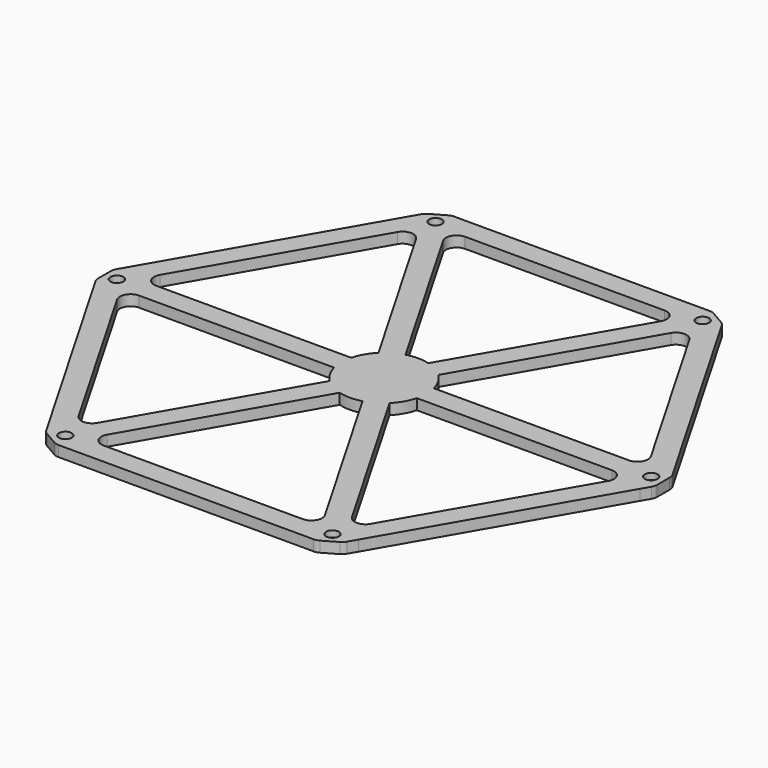
from build123d import *

# Parameters (mm, degrees)
F0_R     = 3
F1_DEPTH = 5
F2_DEPTH = 2
F3_R     = 5
F4_R     = 5
F0_R_2   = 15
F5_DEPTH = 5
F6_DEPTH = 5
F7_DEPTH = 3


# Not quite as in the source:
# - a feature names something its author has since deleted; it is built from what else it names


with BuildPart() as f1:
    # F0 (on Top) → F1 (new body)
    with BuildSketch(Plane.XY):
        Polygon((55.3523313466, 115.8730502097), (-55.3523313466, 115.8730502097), (-61.1258340385, 115.8730502097), (-69.7860880763, 110.8730502097), (-72.6728394223, 105.8730502097), (-128.0251707689, 10), (-130.9119221148, 5), (-130.9119221148, -5), (-128.0251707689, -10), (-72.6728394223, -105.8730502097), (-69.7860880763, -110.8730502097), (-61.1258340385, -115.8730502097), (-55.3523313466, -115.8730502097), (55.3523313466, -115.8730502097), (61.1258340385, -115.8730502097), (69.7860880763, -110.8730502097), (72.6728394223, -105.8730502097), (128.0251707689, -10), (130.9119221148, -5), (130.9119221148, 5), (128.0251707689, 10), (72.6728394223, 105.8730502097), (69.7860880763, 110.8730502097), (61.1258340385, 115.8730502097), align=None)
        with Locations((-62.5692097115, -108.3730502097)):
            Circle(F0_R, mode=Mode.SUBTRACT)
        with Locations((62.5692097115, -108.3730502097)):
            Circle(F0_R, mode=Mode.SUBTRACT)
        with Locations((-125.1384194229, 0)):
            Circle(F0_R, mode=Mode.SUBTRACT)
        Polygon((-119.364916731, -5), (-119.364916731, 0), (-119.364916731, 5), (-64.0125853844, 100.8730502097), (-59.6824583655, 103.3730502097), (-55.3523313466, 105.8730502097), (55.3523313466, 105.8730502097), (59.6824583655, 103.3730502097), (64.0125853844, 100.8730502097), (119.364916731, 5), (119.364916731, 0), (119.364916731, -5), (64.0125853844, -100.8730502097), (59.6824583655, -103.3730502097), (55.3523313466, -105.8730502097), (-55.3523313466, -105.8730502097), (-59.6824583655, -103.3730502097), (-64.0125853844, -100.8730502097), align=None, mode=Mode.SUBTRACT)
        with Locations((-62.5692097115, 108.3730502097)):
            Circle(F0_R, mode=Mode.SUBTRACT)
        with Locations((125.1384194229, 0)):
            Circle(F0_R, mode=Mode.SUBTRACT)
        with Locations((62.5692097115, 108.3730502097)):
            Circle(F0_R, mode=Mode.SUBTRACT)
        with BuildLine():
            Line((-59.6824583655, 103.3730502097), (-64.0125853844, 100.8730502097))
            Line((-64.0125853844, 100.8730502097), (-14.0125853844, 14.2705098312))
            ThreePointArc((-14.0125853844, 14.2705098312), (-10, 17.3205080757), (-5.3523313466, 19.2705098312))
            Line((-5.3523313466, 19.2705098312), (-55.3523313466, 105.8730502097))
            Line((-55.3523313466, 105.8730502097), (-59.6824583655, 103.3730502097))
        make_face()
        with BuildLine():
            Line((55.3523313466, 105.8730502097), (5.3523313466, 19.2705098312))
            ThreePointArc((5.3523313466, 19.2705098312), (10, 17.3205080757), (14.0125853844, 14.2705098312))
            Line((14.0125853844, 14.2705098312), (64.0125853844, 100.8730502097))
            Line((64.0125853844, 100.8730502097), (59.6824583655, 103.3730502097))
            Line((59.6824583655, 103.3730502097), (55.3523313466, 105.8730502097))
        make_face()
        with BuildLine():
            Line((119.364916731, 5), (19.364916731, 5))
            ThreePointArc((19.364916731, 5), (19.8405939253, 2.5200858497), (20, 0))
            ThreePointArc((20, 0), (19.8405939253, -2.5200858497), (19.364916731, -5))
            Line((19.364916731, -5), (119.364916731, -5))
            Line((119.364916731, -5), (119.364916731, 0))
            Line((119.364916731, 0), (119.364916731, 5))
        make_face()
        with BuildLine():
            ThreePointArc((14.0125853844, -14.2705098312), (10, -17.3205080757), (5.3523313466, -19.2705098312))
            Line((5.3523313466, -19.2705098312), (55.3523313466, -105.8730502097))
            Line((55.3523313466, -105.8730502097), (59.6824583655, -103.3730502097))
            Line((59.6824583655, -103.3730502097), (64.0125853844, -100.8730502097))
            Line((64.0125853844, -100.8730502097), (14.0125853844, -14.2705098312))
        make_face()
        with BuildLine():
            Line((-14.0125853844, -14.2705098312), (-64.0125853844, -100.8730502097))
            Line((-64.0125853844, -100.8730502097), (-59.6824583655, -103.3730502097))
            Line((-59.6824583655, -103.3730502097), (-55.3523313466, -105.8730502097))
            Line((-55.3523313466, -105.8730502097), (-5.3523313466, -19.2705098312))
            ThreePointArc((-5.3523313466, -19.2705098312), (-10, -17.3205080757), (-14.0125853844, -14.2705098312))
        make_face()
        with BuildLine():
            Line((-119.364916731, 5), (-119.364916731, 0))
            Line((-119.364916731, 0), (-119.364916731, -5))
            Line((-119.364916731, -5), (-19.364916731, -5))
            ThreePointArc((-19.364916731, -5), (-20, 0), (-19.364916731, 5))
            Line((-19.364916731, 5), (-119.364916731, 5))
        make_face()
    extrude(amount=F1_DEPTH)

    # F0 (on Top) → F2 (join)
    with BuildSketch(Plane.XY):
        with Locations((-125.1384194229, 0)):
            Circle(F0_R)
        with Locations((-62.5692097115, 108.3730502097)):
            Circle(F0_R)
        with Locations((62.5692097115, 108.3730502097)):
            Circle(F0_R)
        with Locations((125.1384194229, 0)):
            Circle(F0_R)
        with Locations((62.5692097115, -108.3730502097)):
            Circle(F0_R)
        with Locations((-62.5692097115, -108.3730502097)):
            Circle(F0_R)
    extrude(amount=F2_DEPTH)

    # F3
    f3_edges = [f1.edges().sort_by_distance(p)[0] for p in [
        (-130.911922, 5, 2.5),
        (-130.911922, -5, 2.5),
        (-69.786088, -110.87305, 2.5),
        (-61.125834, -115.87305, 2.5),
        (61.125834, -115.87305, 2.5),
        (69.786088, -110.87305, 2.5),
        (130.911922, -5, 2.5),
        (130.911922, 5, 2.5),
        (69.786088, 110.87305, 2.5),
        (61.125834, 115.87305, 2.5),
        (-61.125834, 115.87305, 2.5),
        (-69.786088, 110.87305, 2.5),
    ]]
    fillet(f3_edges, radius=F3_R)

    # F4
    f4_edges = [f1.edges().sort_by_distance(p)[0] for p in [
        (-64.012585, 100.87305, 2.5),
        (-55.352331, 105.87305, 2.5),
        (55.352331, 105.87305, 2.5),
        (64.012585, 100.87305, 2.5),
        (119.364917, 5, 2.5),
        (119.364917, -5, 2.5),
        (64.012585, -100.87305, 2.5),
        (55.352331, -105.87305, 2.5),
        (-55.352331, -105.87305, 2.5),
        (-64.012585, -100.87305, 2.5),
        (-119.364917, -5, 2.5),
        (-119.364917, 5, 2.5),
    ]]
    fillet(f4_edges, radius=F4_R)

    # F0 (on Top) → F5 (join)
    with BuildSketch(Plane.XY):
        with BuildLine():
            ThreePointArc((-14.0125853844, 14.2705098312), (-17.3205080757, 10), (-19.364916731, 5))
            ThreePointArc((-19.364916731, 5), (-20, 0), (-19.364916731, -5))
            ThreePointArc((-19.364916731, -5), (-17.3205080757, -10), (-14.0125853844, -14.2705098312))
            ThreePointArc((-14.0125853844, -14.2705098312), (-10, -17.3205080757), (-5.3523313466, -19.2705098312))
            ThreePointArc((-5.3523313466, -19.2705098312), (0, -20), (5.3523313466, -19.2705098312))
            ThreePointArc((5.3523313466, -19.2705098312), (10, -17.3205080757), (14.0125853844, -14.2705098312))
            ThreePointArc((14.0125853844, -14.2705098312), (17.3205080757, -10), (19.364916731, -5))
            ThreePointArc((19.364916731, -5), (19.8405939253, -2.5200858497), (20, 0))
            ThreePointArc((20, 0), (19.8405939253, 2.5200858497), (19.364916731, 5))
            ThreePointArc((19.364916731, 5), (17.3205080757, 10), (14.0125853844, 14.2705098312))
            ThreePointArc((14.0125853844, 14.2705098312), (10, 17.3205080757), (5.3523313466, 19.2705098312))
            ThreePointArc((5.3523313466, 19.2705098312), (0, 20), (-5.3523313466, 19.2705098312))
            ThreePointArc((-5.3523313466, 19.2705098312), (-10, 17.3205080757), (-14.0125853844, 14.2705098312))
        make_face()
        Circle(F0_R_2, mode=Mode.SUBTRACT)
    extrude(amount=F5_DEPTH)

    # F0 (on Top) → F6 (join)
    with BuildSketch(Plane.XY):
        Circle(F0_R_2)
    extrude(amount=F6_DEPTH)

    # F0 (on Top) → F7 (cut)
    with BuildSketch(Plane.XY):
        Circle(F0_R_2)
    extrude(amount=F7_DEPTH, mode=Mode.SUBTRACT)


solid = f1.part
